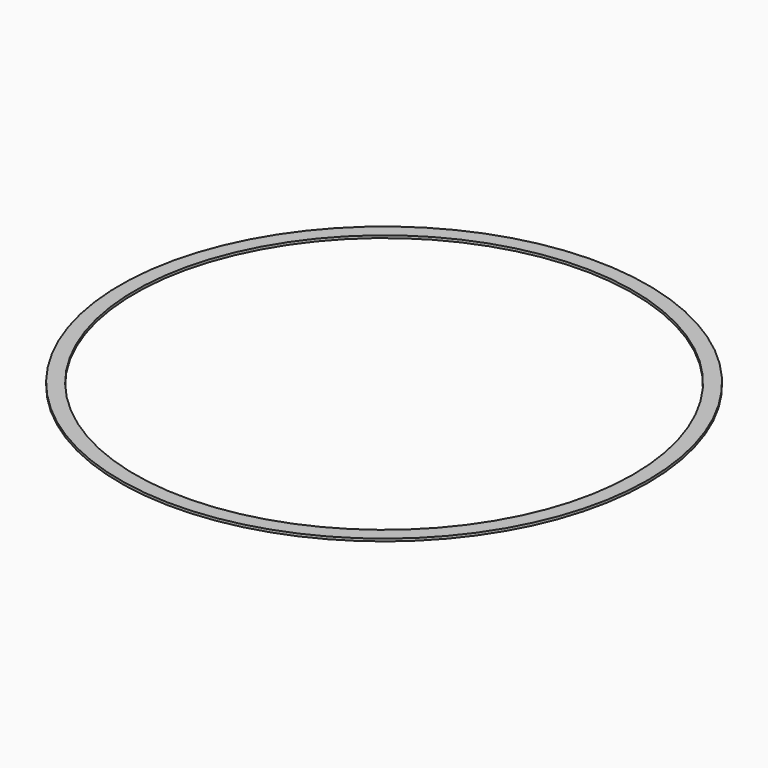
from build123d import *

# Parameters (mm, degrees)
F0_R     = 450.52869
F0_R_2   = 425.12869
F1_DEPTH = 4.2333333333


# Not quite as in the source:
# - a length typed as a fraction of an inch, garbled in the dataset ("3 / 203.2 mm" for 3/8 in), is restored


with BuildPart() as f1:
    # F0 (on Top) → F1 (new body)
    with BuildSketch(Plane.XY):
        Circle(F0_R)
        Circle(F0_R_2, mode=Mode.SUBTRACT)
    extrude(amount=F1_DEPTH)


solid = f1.part
